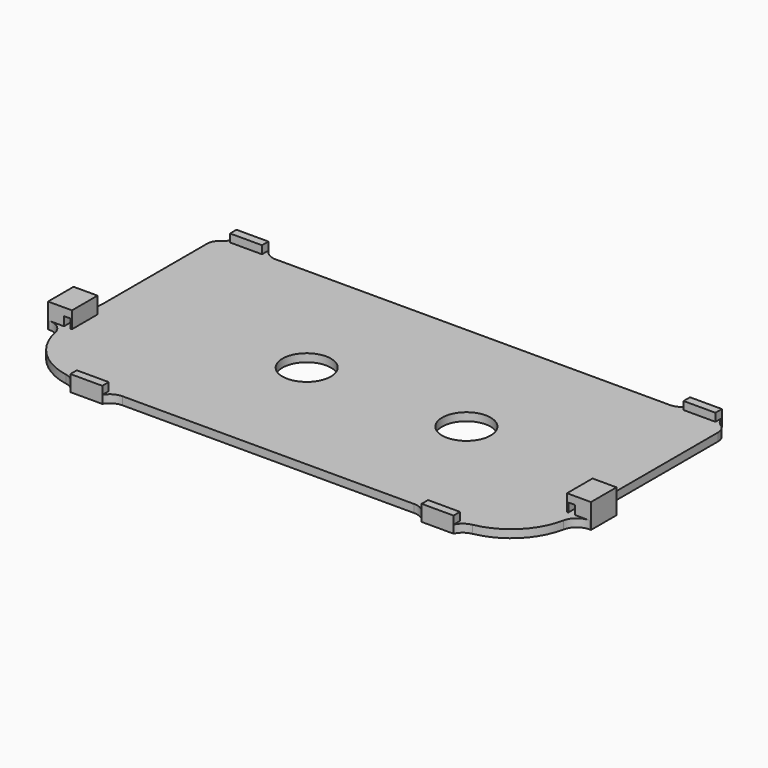
from build123d import *

# Parameters (mm, degrees)
F0_W         = 101.6
F0_H         = 50.8
F0_R         = 1.905
F1_DEPTH     = 1.5875
F3_R         = 12.7
F4_R         = 2.54
F2_R         = 4.826
F2_R_2       = 1.905
F5_DEPTH     = 3.175
F6_W         = 6.35
F6_H         = 1.5875
F7_DEPTH     = 1.6002
F8_W         = 6.35
F8_H         = 1.5875
F9_DEPTH     = 1.6002
F10_W        = 6.35
F10_H        = 1.5875
F11_DEPTH    = 3.175
F12_W        = 6.35
F12_H        = 1.5875
F13_DEPTH    = 3.175
F14_W        = 6.35
F14_H        = 1.6002
F15_DEPTH    = 1.5875
F14_W_2      = 3.175
F14_H_2      = 6.35
F16_DEPTH    = 3.302
F17_W        = 6.35
F17_H        = 1.524
F18_DEPTH    = 1.5875
F19_W        = 6.35
F19_H        = 1.524
F20_DEPTH    = 1.5875
F21_T1_DEPTH = 1.5875
F22_W        = 0.254
F22_H        = 6.35
F23_DEPTH    = 2.032
F24_W        = 0.254
F24_H        = 6.35
F25_DEPTH    = 2.032


# Not quite as in the source:
# - a fillet or chamfer that OpenCascade refuses, or shapes differently, is made with other operations: its cross-section is extruded or revolved along the edge and cut away or added


with BuildPart() as f1:
    # F0 (on Top) → F1 (new body)
    with BuildSketch(Plane.XY):
        Rectangle(F0_W, F0_H)
        with Locations((-12.7, 0)):
            Circle(F0_R, mode=Mode.SUBTRACT)
        with Locations((19.05, 0)):
            Circle(F0_R, mode=Mode.SUBTRACT)
    extrude(amount=F1_DEPTH)

    # F3
    f3_edges = [f1.edges().sort_by_distance(p)[0] for p in [
        (-50.8, -25.4, 0.79375),
        (50.8, -25.4, 0.79375),
    ]]
    fillet(f3_edges, radius=F3_R)

    # F4
    f4_edges = [f1.edges().sort_by_distance(p)[0] for p in [
        (-50.8, 25.4, 0.79375),
        (50.8, 25.4, 0.79375),
    ]]
    fillet(f4_edges, radius=F4_R)

    # F2 (on face) → F5 (cut)
    with BuildSketch(Plane.XY.offset(1.5875)):
        with Locations((-12.7, 0)):
            Circle(F2_R)
        with Locations((-12.7, 0)):
            Circle(F2_R_2, mode=Mode.SUBTRACT)
        with Locations((19.05, 0)):
            Circle(F2_R)
        with Locations((19.05, 0)):
            Circle(F2_R_2, mode=Mode.SUBTRACT)
    extrude(amount=-F5_DEPTH, mode=Mode.SUBTRACT)

    # F6 (on face) → F7 (join)
    with BuildSketch(Plane(origin=(0, 25.4, 0), x_dir=(-1, 0, 0), z_dir=(0, 1, 0))):
        with Locations((-45.085, 0.79375)):
            Rectangle(F6_W, F6_H)
        with Locations((45.085, 0.79375)):
            Rectangle(F6_W, F6_H)
    extrude(amount=F7_DEPTH)

    # F8 (on face) → F9 (join)
    with BuildSketch(Plane.XZ.offset(25.4)):
        with Locations((34.925, 0.79375)):
            Rectangle(F8_W, F8_H)
        with Locations((-34.925, 0.79375)):
            Rectangle(F8_W, F8_H)
    extrude(amount=F9_DEPTH)

    # F10 (on face) → F11 (join)
    with BuildSketch(Plane(origin=(-50.8, 0, 0), x_dir=(0, -1, 0), z_dir=(-1, 0, 0))):
        with Locations((9.525, 0.79375)):
            Rectangle(F10_W, F10_H)
    extrude(amount=F11_DEPTH)

    # F12 (on face) → F13 (join)
    with BuildSketch(Plane.YZ.offset(50.8)):
        with Locations((-9.525, 0.79375)):
            Rectangle(F12_W, F12_H)
    extrude(amount=F13_DEPTH)

    # F14 (on face) → F15 (join)
    with BuildSketch(Plane.XY.offset(1.5875)):
        with Locations((45.085, 26.2001)):
            Rectangle(F14_W, F14_H)
        with Locations((34.925, -26.2001)):
            Rectangle(F14_W, F14_H)
        with Locations((-34.925, -26.2001)):
            Rectangle(F14_W, F14_H)
        with Locations((-45.085, 26.2001)):
            Rectangle(F14_W, F14_H)
    extrude(amount=F15_DEPTH)

    # F14 (on face) → F16 (join)
    with BuildSketch(Plane.XY.offset(1.5875)):
        with Locations((52.3875, -9.525)):
            Rectangle(F14_W_2, F14_H_2)
        with Locations((-52.3875, -9.525)):
            Rectangle(F14_W_2, F14_H_2)
    extrude(amount=F16_DEPTH)

    # F17 (on face) → F18 (join)
    with BuildSketch(Plane.YZ.offset(-50.8)):
        with Locations((-9.525, 4.1275)):
            Rectangle(F17_W, F17_H)
    extrude(amount=F18_DEPTH)

    # F19 (on face) → F20 (join)
    with BuildSketch(Plane(origin=(50.8, 0, 0), x_dir=(0, -1, 0), z_dir=(-1, 0, 0))):
        with Locations((9.525, 4.1275)):
            Rectangle(F19_W, F19_H)
    extrude(amount=F20_DEPTH)

    # F21: fillet of radius 3.175 on 12 edges, made by hand

    # F21_s2 → F21_t1 (join)
    with BuildSketch(Plane.XY):
        with BuildLine():
            ThreePointArc((-28.9930759967, -25.4), (-30.5869133472, -25.8290379646), (-31.75, -27.0002))
            Line((-31.75, -27.0002), (-31.75, -25.4))
            Line((-31.75, -25.4), (-28.9930759967, -25.4))
        make_face()
        with BuildLine():
            ThreePointArc((-38.1, -27.0002), (-39.0345990401, -25.8098604937), (-40.4140641084, -25.1873979396))
            ThreePointArc((-40.4140641084, -25.1873979396), (-39.2619049374, -25.3467377974), (-38.1, -25.4))
            Line((-38.1, -25.4), (-38.1, -27.0002))
        make_face()
        with BuildLine():
            ThreePointArc((-50.5434078933, -15.24), (-51.6462135525, -13.4156555752), (-53.6542598667, -12.7))
            Line((-53.6542598667, -12.7), (-50.8, -12.7))
            ThreePointArc((-50.8, -12.7), (-50.7356891432, -13.9764638175), (-50.5434078933, -15.24))
        make_face()
        with BuildLine():
            ThreePointArc((-53.975, -6.35), (-51.7299359697, -5.4200640303), (-50.8, -3.175))
            Line((-50.8, -3.175), (-50.8, -6.35))
            Line((-50.8, -6.35), (-53.975, -6.35))
        make_face()
        with BuildLine():
            ThreePointArc((-49.6405789052, 24.9920417178), (-48.7499512331, 25.8583913172), (-48.26, 27.0002))
            Line((-48.26, 27.0002), (-48.26, 25.4))
            ThreePointArc((-48.26, 25.4), (-48.9797965118, 25.2958762246), (-49.6405789052, 24.9920417178))
        make_face()
        with BuildLine():
            ThreePointArc((-41.91, 27.0002), (-40.7469133472, 25.8290379646), (-39.1530759967, 25.4))
            Line((-39.1530759967, 25.4), (-41.91, 25.4))
            Line((-41.91, 25.4), (-41.91, 27.0002))
        make_face()
        with BuildLine():
            ThreePointArc((48.26, 27.0002), (48.7499512331, 25.8583913172), (49.6405789052, 24.9920417178))
            ThreePointArc((49.6405789052, 24.9920417178), (48.9797965118, 25.2958762246), (48.26, 25.4))
            Line((48.26, 25.4), (48.26, 27.0002))
        make_face()
        with BuildLine():
            ThreePointArc((39.1530759967, 25.4), (40.7469133472, 25.8290379646), (41.91, 27.0002))
            Line((41.91, 27.0002), (41.91, 25.4))
            Line((41.91, 25.4), (39.1530759967, 25.4))
        make_face()
        with BuildLine():
            ThreePointArc((50.8, -3.175), (51.7299359697, -5.4200640303), (53.975, -6.35))
            Line((53.975, -6.35), (50.8, -6.35))
            Line((50.8, -6.35), (50.8, -3.175))
        make_face()
        with BuildLine():
            ThreePointArc((53.6542598667, -12.7), (51.6462135525, -13.4156555752), (50.5434078933, -15.24))
            ThreePointArc((50.5434078933, -15.24), (50.7356891432, -13.9764638175), (50.8, -12.7))
            Line((50.8, -12.7), (53.6542598667, -12.7))
        make_face()
        with BuildLine():
            ThreePointArc((40.4140641084, -25.1873979396), (39.0345990401, -25.8098604937), (38.1, -27.0002))
            Line((38.1, -27.0002), (38.1, -25.4))
            ThreePointArc((38.1, -25.4), (39.2619049374, -25.3467377974), (40.4140641084, -25.1873979396))
        make_face()
        with BuildLine():
            ThreePointArc((31.75, -27.0002), (30.5869133472, -25.8290379646), (28.9930759967, -25.4))
            Line((28.9930759967, -25.4), (31.75, -25.4))
            Line((31.75, -25.4), (31.75, -27.0002))
        make_face()
    extrude(amount=F21_T1_DEPTH)

    # F22 (on face) → F23 (join)
    with BuildSketch(Plane(origin=(0, 0, 3.3655), x_dir=(1, 0, 0), z_dir=(0, 0, -1))):
        with Locations((49.3395, 9.525)):
            Rectangle(F22_W, F22_H)
    extrude(amount=F23_DEPTH)

    # F24 (on face) → F25 (join)
    with BuildSketch(Plane(origin=(0, 0, 3.3655), x_dir=(1, 0, 0), z_dir=(0, 0, -1))):
        with Locations((-49.3395, 9.525)):
            Rectangle(F24_W, F24_H)
    extrude(amount=F25_DEPTH)


solid = f1.part
